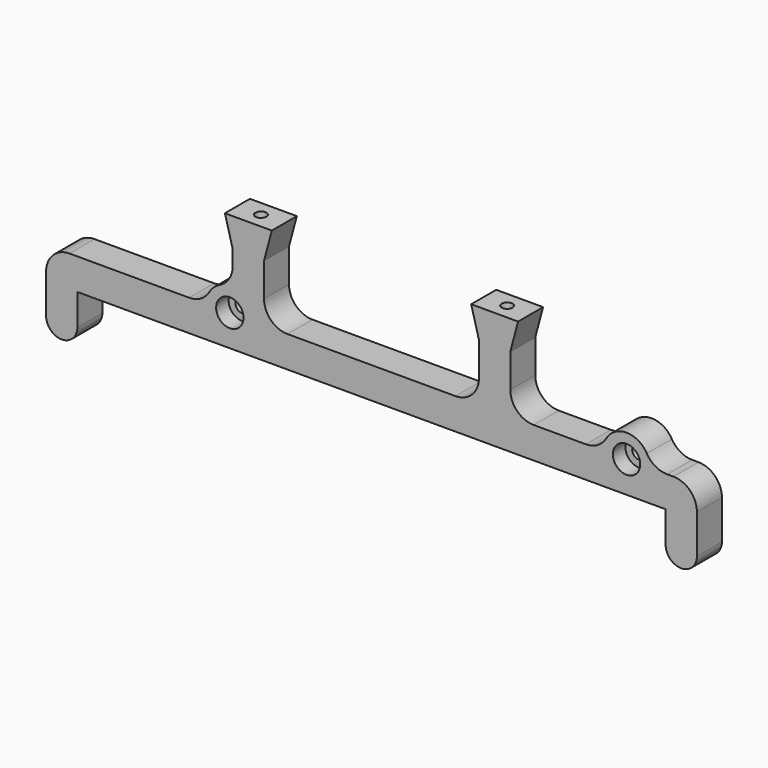
from build123d import *

# Parameters (mm, degrees)
F0_R     = 1.75
F1_DEPTH = 8
F2_R     = 6
F3_R     = 3.5
F4_DEPTH = 4
F5_R     = 1.4
F6_DEPTH = 15
F7_R     = 1.4
F8_DEPTH = 15


# Not quite as in the source:
# - a feature names something its author has since deleted; it is built from what else it names


with BuildPart() as f1:
    # F0 (on Front) → F1 (new body)
    with BuildSketch(Plane.XZ):
        with BuildLine():
            Line((-75.25, 0), (0, 0))
            Line((0, 0), (75.25, 0))
            Line((75.25, 0), (75.25, -8))
            ThreePointArc((75.25, -8), (79.25, -12), (83.25, -8))
            Line((83.25, -8), (83.25, 8))
            Line((83.25, 8), (71.25, 8))
            ThreePointArc((71.25, 8), (65.25, 14), (59.25, 8))
            Line((59.25, 8), (35.5, 8))
            Line((35.5, 8), (35.5, 22.5358983849))
            Line((35.5, 22.5358983849), (35.5, 30))
            Line((35.5, 30), (27.5, 30))
            Line((27.5, 30), (27.5, 22.5358983849))
            Line((27.5, 22.5358983849), (27.5, 8))
            Line((27.5, 8), (0, 8))
            Line((0, 8), (-27.5, 8))
            Line((-27.5, 8), (-27.5, 22.5358983849))
            Line((-27.5, 22.5358983849), (-27.5, 30))
            Line((-27.5, 30), (-35.5, 30))
            Line((-35.5, 30), (-35.5, 22.5358983849))
            Line((-35.5, 22.5358983849), (-35.5, 13.9529404499))
            ThreePointArc((-35.5, 13.9529404499), (-40.2186269666, 12.5), (-42.25, 8))
            Line((-42.25, 8), (-83.25, 8))
            Line((-83.25, 8), (-83.25, -8))
            ThreePointArc((-83.25, -8), (-79.25, -12), (-75.25, -8))
            Line((-75.25, -8), (-75.25, 0))
        make_face()
        with Locations((-36.25, 8)):
            Circle(F0_R, mode=Mode.SUBTRACT)
        with Locations((65.25, 8)):
            Circle(F0_R, mode=Mode.SUBTRACT)
        Polygon((-37.5, 30), (-35.5, 22.5358983849), (-35.5, 30), align=None)
        Polygon((-25.5, 30), (-27.5, 30), (-27.5, 22.5358983849), align=None)
        Polygon((27.5, 22.5358983849), (27.5, 30), (25.5, 30), align=None)
        Polygon((35.5, 30), (35.5, 22.5358983849), (37.5, 30), align=None)
    extrude(amount=F1_DEPTH)

    # F2
    f2_edges = [f1.edges().sort_by_distance(p)[0] for p in [
        (59.25, -4, 8),
        (71.25, -4, 8),
        (83.25, -4, 8),
        (-83.25, -4, 8),
        (-35.5, -4, 13.95294),
        (-27.5, -4, 8),
        (27.5, -4, 8),
        (35.5, -4, 8),
        (-42.25, -4, 8),
    ]]
    fillet(f2_edges, radius=F2_R)

    # F3 (on face) → F4 (cut)
    with BuildSketch(Plane.XZ.offset(8)):
        with Locations((-36.25, 8)):
            Circle(F3_R)
        with Locations((65.25, 8)):
            Circle(F3_R)
    extrude(amount=-F4_DEPTH, mode=Mode.SUBTRACT)

    # F5 (on face) → F6 (cut)
    with BuildSketch(Plane.XY.offset(30)):
        with Locations((-31.5, -4)):
            Circle(F5_R)
    extrude(amount=-F6_DEPTH, mode=Mode.SUBTRACT)

    # F7 (on face) → F8 (cut)
    with BuildSketch(Plane.XY.offset(30)):
        with Locations((31.5, -4)):
            Circle(F7_R)
    extrude(amount=-F8_DEPTH, mode=Mode.SUBTRACT)


solid = f1.part
